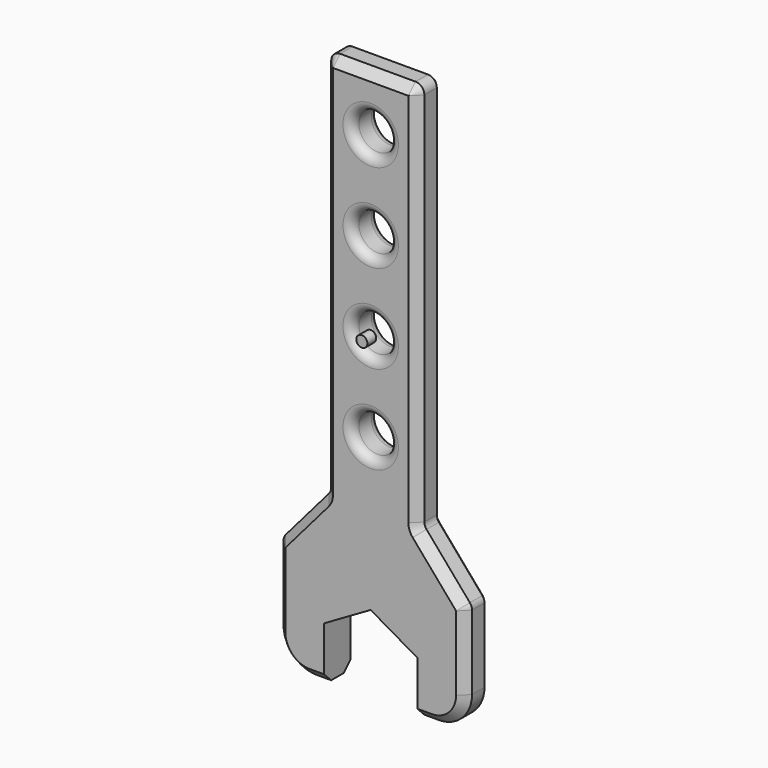
from build123d import *

# Parameters (mm, degrees)
F1_DEPTH     = 1.5
F2_R         = 1.7
F3_DEPTH     = 3.001
F4_R         = 0.8
F5_R         = 3
F6_SIZE      = 0.79999
F7_TEXT_SIZE = 8.3202526955
F8_DEPTH     = 0.8
F9_R         = 0.5
F10_DEPTH    = 1


# Not quite as in the source:
# - a fillet or chamfer is up to 0.001 mm smaller than in the source, because OpenCascade refuses the exact size
# - a feature names something its author has since deleted; it is built from what else it names
# - Text() gives the source's letters only with a copy of the font that has no kerning and outlines rounded to 1/6400 em; it was checked with that copy


with BuildPart() as f1:
    # F0 (on Front) → F1 (new body, symmetric)
    with BuildSketch(Plane.XZ):
        Polygon((2.1, 3.6373066959), (4.2, 2.4248711306), (4.2, -2.4248711306), (8.5, -2.4248711306), (8.5, 7.5751288694), (4.2, 12.5751288694), (4.2, 47.5751288694), (0, 47.5751288694), (-4.2, 47.5751288694), (-4.2, 12.5751288694), (-8.5, 7.5751288694), (-8.5, -2.4248711306), (-4.2, -2.4248711306), (-4.2, 2.4248711306), (0, 4.8497422612), align=None)
    extrude(amount=F1_DEPTH, both=True)

    # F2 (on face) → F3 (cut, through all)
    with BuildSketch(Plane.XZ.offset(1.5)):
        with Locations((0, 42.5751288694)):
            Circle(F2_R)
        with Locations((0, 34.5751288694)):
            Circle(F2_R)
        with Locations((0, 26.5751288694)):
            Circle(F2_R)
        with Locations((0, 18.5751288694)):
            Circle(F2_R)
    extrude(amount=-F3_DEPTH, mode=Mode.SUBTRACT)

    # F4
    f4_edges = [f1.edges().sort_by_distance(p)[0] for p in [
        (-1.7, 1.5, 18.575129),
        (-1.7, 1.5, 42.575129),
        (-1.7, 1.5, 34.575129),
        (-1.7, 1.5, 26.575129),
        (-1.7, -1.5, 18.575129),
        (-1.7, -1.5, 26.575129),
        (-1.7, -1.5, 34.575129),
        (-1.7, -1.5, 42.575129),
        (-4.2, 0, 47.575129),
        (4.2, 0, 47.575129),
        (8.5, 0, 7.575129),
        (-4.2, 0, 12.575129),
        (-8.5, 0, 7.575129),
        (4.2, 0, 12.575129),
    ]]
    fillet(f4_edges, radius=F4_R)

    # F5
    f5_edges = [f1.edges().sort_by_distance(p)[0] for p in [
        (-8.5, 0, -2.424871),
        (8.5, 0, -2.424871),
    ]]
    fillet(f5_edges, radius=F5_R)

    # F6 (size 0.8 in the source; OpenCascade refuses exactly that, so slightly less here)
    f6_edges = [f1.edges().sort_by_distance(p)[0] for p in [
        (6.35, 1.5, 10.075129),
        (-8.5, -1.5, 3.926785),
        (8.5, 1.5, 3.926785),
        (7.62132, 1.5, -1.546191),
        (8.45008, 1.5, 7.556615),
        (4.85, 1.5, -2.424871),
        (4.24992, 1.5, 12.593642),
        (4.2, 1.5, 29.823473),
        (3.965685, 1.5, 47.340814),
        (0, 1.5, 47.575129),
        (-4.85, 1.5, -2.424871),
        (-3.965685, 1.5, 47.340814),
        (-7.62132, 1.5, -1.546191),
        (-4.2, 1.5, 29.823473),
        (-8.5, 1.5, 3.926785),
        (-4.24992, 1.5, 12.593642),
        (-8.45008, 1.5, 7.556615),
        (-6.35, 1.5, 10.075129),
        (8.5, -1.5, 3.926785),
        (7.62132, -1.5, -1.546191),
        (8.45008, -1.5, 7.556615),
        (4.85, -1.5, -2.424871),
        (6.35, -1.5, 10.075129),
        (4.24992, -1.5, 12.593642),
        (4.2, -1.5, 29.823473),
        (3.965685, -1.5, 47.340814),
        (0, -1.5, 47.575129),
        (-4.85, -1.5, -2.424871),
        (-3.965685, -1.5, 47.340814),
        (-7.62132, -1.5, -1.546191),
        (-4.2, -1.5, 29.823473),
        (-4.24992, -1.5, 12.593642),
        (-8.45008, -1.5, 7.556615),
        (-6.35, -1.5, 10.075129),
    ]]
    chamfer(f6_edges, length=F6_SIZE)

    # F7 (on face) → F8 (cut)
    with BuildSketch(Plane(origin=(0, 1.5, 0), x_dir=(-1, 0, 0), z_dir=(0, 1, 0))):
        with Locations((-2.4706993473, 5.8379715101)):
            Text('8', F7_TEXT_SIZE, font='Open Sans', text_align=(TextAlign.LEFT, TextAlign.BOTTOM))
    extrude(amount=-F8_DEPTH, mode=Mode.SUBTRACT)


with BuildPart() as f10:
    # F9 (on face) → F10 (new body)
    with BuildSketch(Plane.XZ.offset(1.5)):
        with Locations((0, 26.5751288694)):
            Circle(F9_R)
    extrude(amount=F10_DEPTH)


solid = Compound([f1.part, f10.part])
